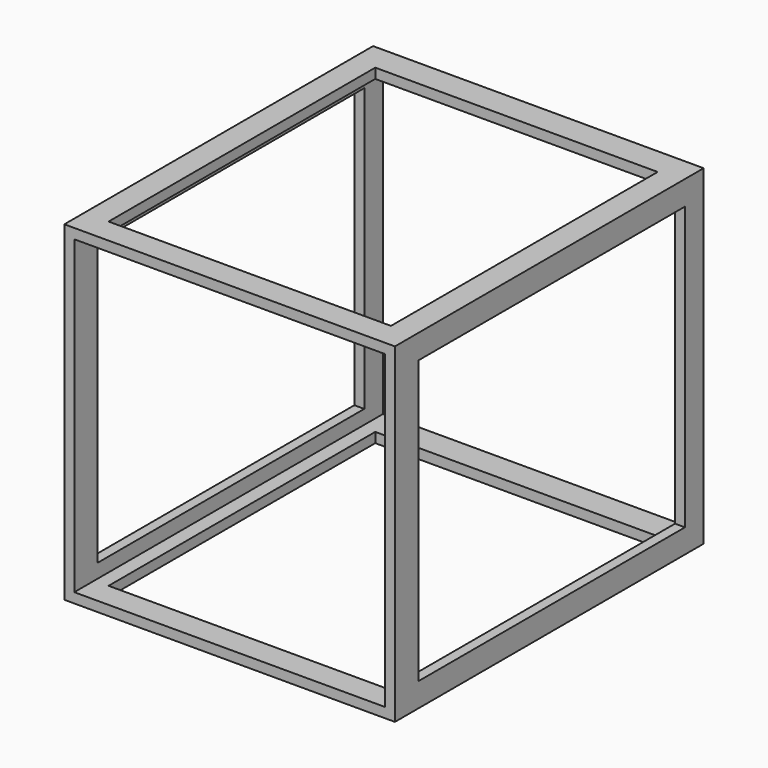
from build123d import *

# Parameters (mm, degrees)
F0_W     = 116.5
F0_H     = 116.5
F0_W_2   = 109.5
F0_H_2   = 109.5
F1_DEPTH = 136
F2_W     = 99.5149090886
F2_H     = 117.4702011049
F3_DEPTH = 186
F4_W     = 117.4702011049
F4_H     = 99.5149090886
F5_DEPTH = 134.2


# Not quite as in the source:
# - a feature of the source that left no trace in its solid (it failed there, or was rolled back) is left out


with BuildPart() as f1:
    # F0 (on Front) → F1 (new body)
    with BuildSketch(Plane.XZ):
        Rectangle(F0_W, F0_H)
        Rectangle(F0_W_2, F0_H_2, mode=Mode.SUBTRACT)
    extrude(amount=F1_DEPTH)

    # F2 (on face) → F3 (cut)
    with BuildSketch(Plane(origin=(0, 0, -58.25), x_dir=(1, 0, 0), z_dir=(0, 0, -1))):
        with Locations((0, 68.3887079358)):
            Rectangle(F2_W, F2_H)
    extrude(amount=-F3_DEPTH, mode=Mode.SUBTRACT)

    # F4 (on face) → F5 (cut)
    with BuildSketch(Plane.YZ.offset(58.25)):
        with Locations((-66.9774990529, -0.0578425825)):
            Rectangle(F4_W, F4_H)
    extrude(amount=-F5_DEPTH, mode=Mode.SUBTRACT)


solid = f1.part
